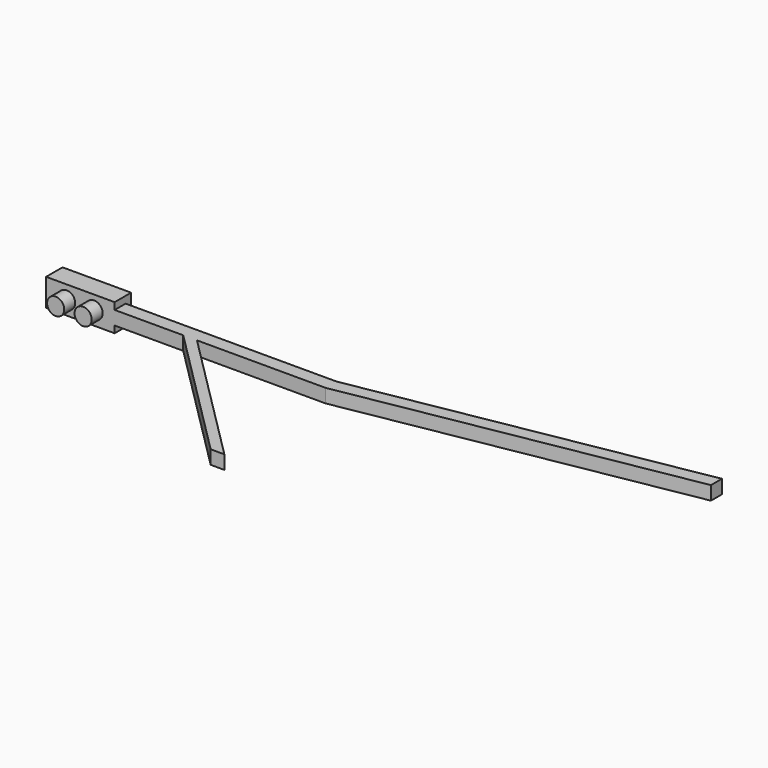
from build123d import *

# Parameters (mm, degrees)
F0_W          = 30.7596123494
F0_H          = 2
F1_DEPTH      = 2
F2_DEPTH      = 3
F2_DEPTH_BACK = 1
F4_DEPTH      = 2
F6_DEPTH      = 2


# Not quite as in the source:
# - a feature names something its author has since deleted; it is built from what else it names


with BuildPart() as f1:
    # F0 (on Top) → F1 (new body)
    with BuildSketch(Plane.XY):
        Polygon((40.7596123494, 2), (40.7596123494, 0), (90, 8.6824088833), (90, 10.6824088833), align=None)
        with Locations((25.3798061747, 1)):
            Rectangle(F0_W, F0_H)
    extrude(amount=F1_DEPTH)

    # F0 (on Top) → F2 (join, two sides)
    with BuildSketch(Plane.XY) as f2_sk:
        Polygon((0, 3), (0, 0), (10, 0), (10, 2), (10, 3), align=None)
    extrude(amount=F2_DEPTH)
    extrude(f2_sk.sketch, amount=-F2_DEPTH_BACK)

    # F3 (on face) → F4 (join)
    with BuildSketch(Plane.XZ):
        with BuildLine():
            ThreePointArc((1.75, 1), (3, -0.25), (4.25, 1))
            Line((4.25, 1), (1.75, 1))
        make_face()
        with BuildLine():
            Line((1.75, 1), (4.25, 1))
            ThreePointArc((4.25, 1), (3, 2.25), (1.75, 1))
        make_face()
        with BuildLine():
            ThreePointArc((8.25, 1), (7, 2.25), (5.75, 1))
            Line((5.75, 1), (8.25, 1))
        make_face()
        with BuildLine():
            Line((8.25, 1), (5.75, 1))
            ThreePointArc((5.75, 1), (7, -0.25), (8.25, 1))
        make_face()
    extrude(amount=F4_DEPTH)

    # F5 (on Top) → F6 (join)
    with BuildSketch(Plane.XY):
        Polygon((42, -20), (22, 0), (20, 0), (40, -20), align=None)
    extrude(amount=F6_DEPTH)


solid = f1.part
